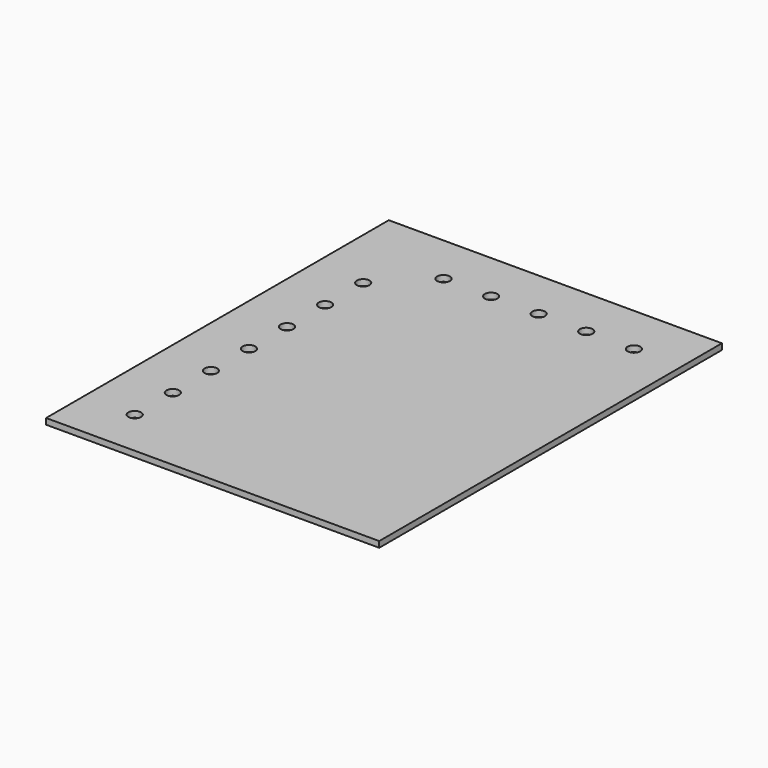
from build123d import *

# Parameters (mm, degrees)
F0_W      = 50.8
F0_H      = 177.8
F1_DEPTH  = 3.175
F3_DEPTH  = 76.2
F5_DEPTH  = 3.175
F7_D      = 6.7564
F7_DEPTH  = 29.21
F7_TIP    = 2.0298273432
F8_W      = 127
F8_H      = 177.8
F8_R      = 3.3782
F9_DEPTH  = 3.175
F10_W     = 247.0957003534
F10_H     = 423.9609837532
F11_DEPTH = 82.55


# Not quite as in the source:
# - an extrude ends at something that could not be found from the text; its depth is read off the source's solid


with BuildPart() as f1:
    # F0 (on Top) → F1 (new body)
    with BuildSketch(Plane.XY):
        Polygon((0, 228.6), (0, 177.8), (50.8, 177.8), (177.8, 177.8), (177.8, 228.6), align=None)
        with Locations((25.4, 88.9)):
            Rectangle(F0_W, F0_H)
    extrude(amount=F1_DEPTH)

    # F2 (on face) → F3 (join)
    with BuildSketch(Plane.XY.offset(3.175)):
        Polygon((3.175, 0), (3.175, 225.425), (177.8, 225.425), (177.8, 228.6), (0, 228.6), (0, 0), align=None)
    extrude(amount=F3_DEPTH)

    # F4 (on face) → F5 (join)
    with BuildSketch(Plane.XY.offset(79.375)):
        Polygon((177.8, 228.6), (0, 228.6), (0, 0), (3.175, 0), (3.175, 225.425), (177.8, 225.425), align=None)
        Polygon((177.8, 177.8), (177.8, 225.425), (3.175, 225.425), (3.175, 0), (50.8, 0), (50.8, 177.8), align=None)
    extrude(amount=F5_DEPTH)

    # F7
    with Locations(Plane.XY.offset(82.55)):
        with Locations((26.9875, 25.4), (26.9875, 50.8), (26.9875, 76.2), (26.9875, 101.6), (26.9875, 127), (26.9875, 152.4), (26.9875, 177.8), (50.8, 201.6125), (76.2, 201.6125), (101.6, 201.6125), (127, 201.6125), (152.4, 201.6125)):
            Hole(F7_D / 2, depth=F7_DEPTH)
            with Locations((0, 0, -(F7_DEPTH + F7_TIP / 2))):  # 118° drill point
                Cone(0, F7_D / 2, F7_TIP, mode=Mode.SUBTRACT)

    # F8 (on face) → F9 (join)
    with BuildSketch(Plane.XY.offset(82.55)):
        with Locations((114.3, 88.9)):
            Rectangle(F8_W, F8_H)
        Polygon((0, 228.6), (0, 0), (50.8, 0), (50.8, 177.8), (177.8, 177.8), (177.8, 228.6), align=None)
        with Locations((26.9875, 25.4)):
            Circle(F8_R, mode=Mode.SUBTRACT)
        with Locations((26.9875, 50.8)):
            Circle(F8_R, mode=Mode.SUBTRACT)
        with Locations((26.9875, 76.2)):
            Circle(F8_R, mode=Mode.SUBTRACT)
        with Locations((26.9875, 101.6)):
            Circle(F8_R, mode=Mode.SUBTRACT)
        with Locations((26.9875, 127)):
            Circle(F8_R, mode=Mode.SUBTRACT)
        with Locations((26.9875, 152.4)):
            Circle(F8_R, mode=Mode.SUBTRACT)
        with Locations((26.9875, 177.8)):
            Circle(F8_R, mode=Mode.SUBTRACT)
        with Locations((50.8, 201.6125)):
            Circle(F8_R, mode=Mode.SUBTRACT)
        with Locations((76.2, 201.6125)):
            Circle(F8_R, mode=Mode.SUBTRACT)
        with Locations((101.6, 201.6125)):
            Circle(F8_R, mode=Mode.SUBTRACT)
        with Locations((127, 201.6125)):
            Circle(F8_R, mode=Mode.SUBTRACT)
        with Locations((152.4, 201.6125)):
            Circle(F8_R, mode=Mode.SUBTRACT)
    extrude(amount=F9_DEPTH)

    # F10 (on Top) → F11 (cut, through all)
    with BuildSketch(Plane.XY):
        with Locations((80.0526309758, 75.9060680866)):
            Rectangle(F10_W, F10_H)
    extrude(amount=F11_DEPTH, mode=Mode.SUBTRACT)


solid = f1.part
